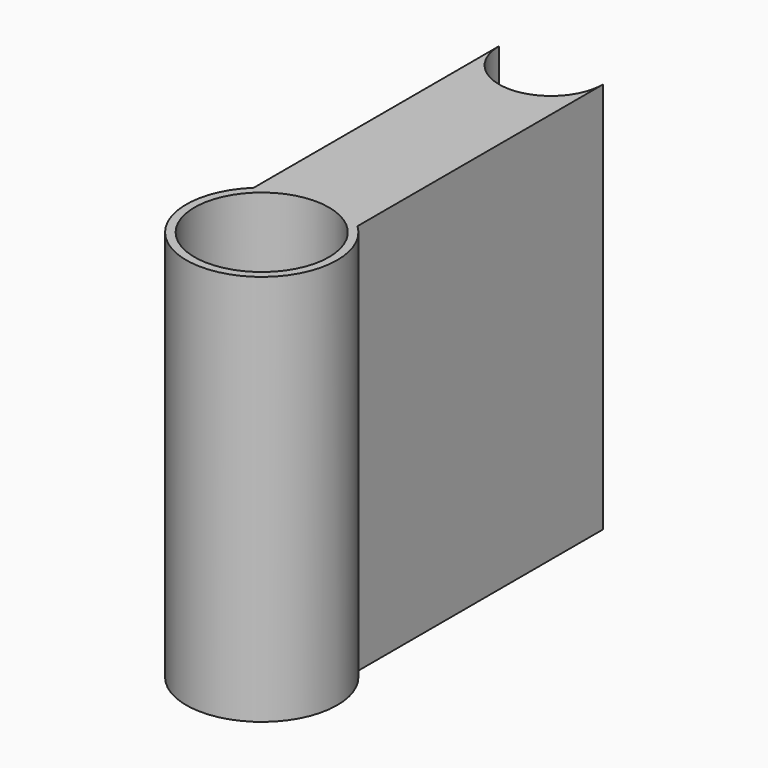
from build123d import *

# Parameters (mm, degrees)
F0_R     = 14.25
F1_DEPTH = 41.5


# Not quite as in the source:
# - ends of sketch curves that miss each other by under 0.0002 mm in the source are joined


with BuildPart() as f1:
    # F0 (on Top) → F1 (new body, symmetric)
    with BuildSketch(Plane.XY):
        with BuildLine():
            ThreePointArc((-11.0000361821, 11.6189157839), (-4.98249e-05, 15.9999999999), (10.9999638179, 11.6189842932))
            Line((10.9999638179, 11.6189842932), (10.9999638179, 76.6189842932))
            ThreePointArc((10.9999638179, 76.6189842932), (3.42546e-05, 65.6189519658), (-10.9999638181, 76.6189157839))
            Line((-10.9999638181, 76.6189157839), (-11.0000361821, 11.6189157839))
        make_face()
        with BuildLine():
            ThreePointArc((-11.0000361821, 11.6189157839), (-6.3245324367, -14.6969483042), (16, 0))
            ThreePointArc((16, 0), (14.6969286092, 6.3245782039), (10.9999638179, 11.6189842932))
            ThreePointArc((10.9999638179, 11.6189842932), (-4.98249e-05, 15.9999999999), (-11.0000361821, 11.6189157839))
        make_face()
        Circle(F0_R, mode=Mode.SUBTRACT)
    extrude(amount=F1_DEPTH, both=True)


solid = f1.part
